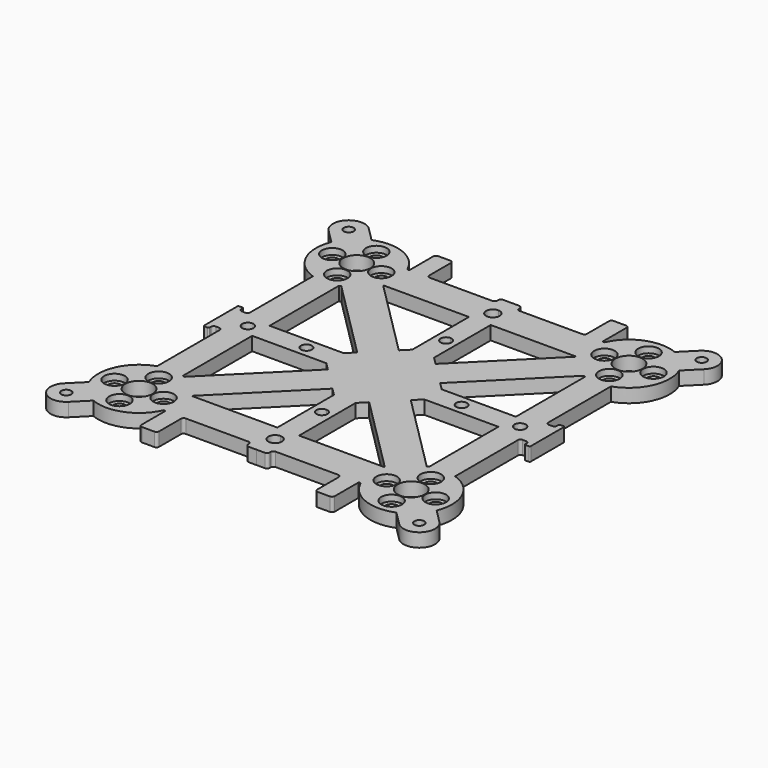
from build123d import *
from build123d import SkipClean  # not in build123d's __all__

# Parameters (mm, degrees)
F0_R     = 1.1
F0_R_2   = 2.5
F0_W     = 3.25
F0_H     = 6
F0_R_3   = 0.9
F1_DEPTH = 2.5
F2_R     = 1.9
F2_R_2   = 1.1
F3_DEPTH = 1.125
F4_W     = 6
F4_H     = 2.5
F5_DEPTH = 21
F6_R     = 0.5
F7_R     = 0.2


with BuildPart() as f1:
    # F0 (on Top) → F1 (new body)
    with BuildSketch(Plane.XY):
        with BuildLine():
            ThreePointArc((-18.0181241326, 22.2607648198), (-17.6306693314, 23.6060970273), (-17.5, 25))
            ThreePointArc((-17.5, 25), (-17.658202653, 26.5323223277), (-18.1261364576, 28))
            ThreePointArc((-18.1261364576, 28), (-22.1801937887, 31.9497261047), (-27.8401980388, 31.9414173697))
            ThreePointArc((-27.8401980388, 31.9414173697), (-30.3033008589, 30.3033008589), (-31.9414173697, 27.8401980388))
            ThreePointArc((-31.9414173697, 27.8401980388), (-31.818156018, 21.8754602717), (-27.3805728112, 17.8878362582))
            ThreePointArc((-27.3805728112, 17.8878362582), (-25, 17.5), (-22.6194271888, 17.8878362582))
            ThreePointArc((-22.6194271888, 17.8878362582), (-22.4392672533, 17.9506987722), (-22.2607648198, 18.0181241326))
            ThreePointArc((-22.2607648198, 18.0181241326), (-19.797428461, 19.5978477084), (-18.1261364576, 22))
            ThreePointArc((-18.1261364576, 22), (-18.0709035062, 22.1298742573), (-18.0181241326, 22.2607648198))
        make_face()
        with Locations((-29.5, 25)):
            Circle(F0_R, mode=Mode.SUBTRACT)
        with Locations((-25, 20.5)):
            Circle(F0_R, mode=Mode.SUBTRACT)
        with Locations((-25, 25)):
            Circle(F0_R_2, mode=Mode.SUBTRACT)
        with Locations((-20.5, 25)):
            Circle(F0_R, mode=Mode.SUBTRACT)
        with Locations((-25, 29.5)):
            Circle(F0_R, mode=Mode.SUBTRACT)
        with BuildLine():
            ThreePointArc((-18.1261364576, 28), (-17.658202653, 26.5323223277), (-17.5, 25))
            ThreePointArc((-17.5, 25), (-17.6306693314, 23.6060970273), (-18.0181241326, 22.2607648198))
            Line((-18.0181241326, 22.2607648198), (-17.7573593129, 22))
            Line((-17.7573593129, 22), (-2, 22))
            Line((-2, 22), (-2, 28))
            Line((-2, 28), (-14.5, 28))
            Line((-14.5, 28), (-17.75, 28))
            Line((-17.75, 28), (-18.1261364576, 28))
        make_face()
        with BuildLine():
            ThreePointArc((-31.9414173697, 27.8401980388), (-30.3033008589, 30.3033008589), (-27.8401980388, 31.9414173697))
            Line((-27.8401980388, 31.9414173697), (-30.374011537, 34.4752308679))
            ThreePointArc((-30.374011537, 34.4752308679), (-29.7453705582, 33.5344031563), (-29.5246212025, 32.4246212025))
            ThreePointArc((-29.5246212025, 32.4246212025), (-31.3148392486, 29.7453705582), (-34.4752308679, 30.374011537))
            Line((-34.4752308679, 30.374011537), (-31.9414173697, 27.8401980388))
        make_face()
        with Locations((-16.125, 31)):
            Rectangle(F0_W, F0_H)
        with BuildLine():
            ThreePointArc((-29.5246212025, 32.4246212025), (-29.7453705582, 33.5344031563), (-30.374011537, 34.4752308679))
            ThreePointArc((-30.374011537, 34.4752308679), (-34.4752308679, 34.4752308679), (-34.4752308679, 30.374011537))
            ThreePointArc((-34.4752308679, 30.374011537), (-31.3148392486, 29.7453705582), (-29.5246212025, 32.4246212025))
        make_face()
        with Locations((-32.4246212025, 32.4246212025)):
            Circle(F0_R_3, mode=Mode.SUBTRACT)
        with BuildLine():
            Line((-2, 28), (-2, 22))
            Line((-2, 22), (-2, 9))
            Line((-2, 9), (-2, 2))
            Line((-2, 2), (-9, 2))
            Line((-9, 2), (-22.6194271888, 2))
            Line((-22.6194271888, 2), (-22.6194271888, 17.8878362582))
            ThreePointArc((-22.6194271888, 17.8878362582), (-25, 17.5), (-27.3805728112, 17.8878362582))
            Line((-27.3805728112, 17.8878362582), (-27.3805728112, 3))
            Line((-27.3805728112, 3), (-29, 3))
            Line((-29, 3), (-29, 4))
            Line((-29, 4), (-30, 4))
            Line((-30, 4), (-30, 0))
            Line((-30, 0), (-26.05, 0))
            ThreePointArc((-26.05, 0), (-25, 1.05), (-23.95, 0))
            Line((-23.95, 0), (-15.25, 0))
            ThreePointArc((-15.25, 0), (-14.25, 1), (-13.25, 0))
            Line((-13.25, 0), (0, 0))
            Line((0, 0), (0, 13.25))
            ThreePointArc((0, 13.25), (-1, 14.25), (0, 15.25))
            Line((0, 15.25), (0, 23.75))
            ThreePointArc((0, 23.75), (-1.25, 25), (0, 26.25))
            Line((0, 26.25), (0, 29.2237700671))
            Line((0, 29.2237700671), (-2, 29.2237700671))
            Line((-2, 29.2237700671), (-2, 28))
        make_face()
        Polygon((-2, 9), (-3.3786796564, 7.6213203436), (-7.6213203436, 3.3786796564), (-9, 2), (-2, 2), align=None)
    extrude(amount=F1_DEPTH)

    # F2 (on face) → F3 (cut)
    with BuildSketch(Plane.XY.offset(2.5)):
        with Locations((-29.5, 25)):
            Circle(F2_R)
        with Locations((-29.5, 25)):
            Circle(F2_R_2, mode=Mode.SUBTRACT)
        with Locations((-25, 29.5)):
            Circle(F2_R)
        with Locations((-25, 29.5)):
            Circle(F2_R_2, mode=Mode.SUBTRACT)
        with Locations((-20.5, 25)):
            Circle(F2_R)
        with Locations((-20.5, 25)):
            Circle(F2_R_2, mode=Mode.SUBTRACT)
        with Locations((-25, 20.5)):
            Circle(F2_R)
        with Locations((-25, 20.5)):
            Circle(F2_R_2, mode=Mode.SUBTRACT)
    extrude(amount=-F3_DEPTH, mode=Mode.SUBTRACT)

    # F4 (on face) → F5 (join)
    with BuildSketch(Plane(origin=(-5.5, 5.5, 0), x_dir=(-0.7071067812, -0.7071067812, 0), z_dir=(-0.7071067812, 0.7071067812, 0))):
        with Locations((0, 1.25)):
            Rectangle(F4_W, F4_H)
    extrude(amount=F5_DEPTH)

    # F6
    f6_edges = [f1.edges().sort_by_distance(p)[0] for p in [
        (-27.380573, 3, 1.25),
        (-29, 3, 1.25),
        (-14.5, 28, 1.25),
        (-14.5, 34, 1.25),
        (-17.75, 34, 1.25),
        (-2, 29.22377, 1.25),
        (-2, 28, 1.25),
    ]]
    fillet(f6_edges, radius=F6_R)

    # F7
    f7_edges = [f1.edges().sort_by_distance(p)[0] for p in [
        (-30, 4, 1.25),
        (-29, 4, 1.25),
    ]]
    fillet(f7_edges, radius=F7_R)

    # F8: F1 across face


with BuildPart() as f1_1:
    add(f1.part, clean=False)
    with SkipClean():  # cleaning this boolean's faces spoils the solid; the shape is the same uncleaned
        add(f1.part.mirror(Plane(origin=(-6.625, 0, 1.25), x_dir=(1, 0, 0), z_dir=(0, -1, 0))), clean=False)

    # F9: F1 across face


with BuildPart() as f1_2:
    add(f1_1.part, clean=False)
    add(f1_1.part.mirror(Plane(origin=(0, 19.5, 1.25), x_dir=(0, 1, 0), z_dir=(1, 0, 0))), clean=False)


solid = f1_2.part
